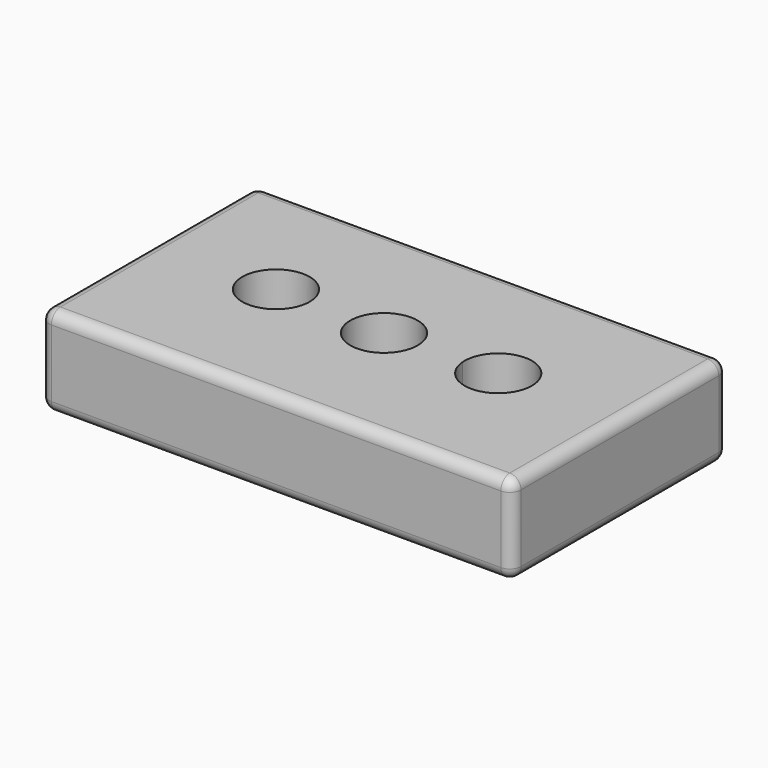
from build123d import *

# Parameters (mm, degrees)
F0_W        = 105
F0_H        = 60
F1_DEPTH    = 20
F2_R        = 2.5
F3_R        = 2.5
F4_R        = 2.5
F5_T1_DEPTH = 23.75
F5_S5_W     = 2.5
F5_S5_H     = 2.5
F5_T6_DEPTH = 2.5
F6_R        = 2.5


# Not quite as in the source:
# - a fillet or chamfer that OpenCascade refuses, or shapes differently, is made with other operations: its cross-section is extruded or revolved along the edge and cut away or added


with BuildPart() as f1:
    # F0 (on Top) → F1 (new body)
    with BuildSketch(Plane.XY):
        Rectangle(F0_W, F0_H)
        with BuildLine():
            ThreePointArc((-17.4192723763, 1.0974504119), (-17.4394815095, 0.547242643), (-17.5, 0))
            ThreePointArc((-17.5, 0), (-32.3990632431, 1.6476581808), (-17.4192723763, 1.0974504119))
        make_face(mode=Mode.SUBTRACT)
        with BuildLine():
            ThreePointArc((-7.5, 0), (0, 7.5), (7.5, 0))
            ThreePointArc((7.5, 0), (0, -7.5), (-7.5, 0))
        make_face(mode=Mode.SUBTRACT)
        with BuildLine():
            ThreePointArc((32.4798090562, 0.5499604379), (25.2549745325, -6.9449901264), (17.5, 0))
            ThreePointArc((17.5, 0), (24.7046435799, 8.0449110021), (32.4798090562, 0.5499604379))
        make_face(mode=Mode.SUBTRACT)
    extrude(amount=F1_DEPTH)

    # F2
    f2_edges = [f1.edges().sort_by_distance(p)[0] for p in [
        (0, -30, 20),
    ]]
    fillet(f2_edges, radius=F2_R)

    # F3
    f3_edges = [f1.edges().sort_by_distance(p)[0] for p in [
        (52.5, 1.25, 20),
        (0, 30, 20),
    ]]
    fillet(f3_edges, radius=F3_R)

    # F4
    f4_edges = [f1.edges().sort_by_distance(p)[0] for p in [
        (-52.5, 0, 20),
    ]]
    fillet(f4_edges, radius=F4_R)

    # F5: fillet of radius 2.5 on 1 edges, made by hand

    # F5_s2 → F5_t1 (cut)
    with BuildSketch(Plane.XY.offset(-6.25)):
        with BuildLine():
            ThreePointArc((50, 30), (51.767766953, 29.267766953), (52.5, 27.5))
            Line((52.5, 27.5), (52.5, 30))
            Line((52.5, 30), (50, 30))
        make_face()
    extrude(amount=F5_T1_DEPTH, mode=Mode.SUBTRACT)


with BuildPart() as f5_tool4:
    # F5_s5 → F5_t6 (new body)
    with BuildSketch(Plane.XZ.offset(-27.5)):
        with Locations((51.25, 18.75)):
            Rectangle(F5_S5_W, F5_S5_H)
    extrude(amount=-F5_T6_DEPTH)

    # F5_s7 → F5_t8 (revolve, cut)
    with BuildSketch(Plane(origin=(50, 27.5, 17.5), x_dir=(-0.7071067812, 0, -0.7071067812), z_dir=(0.7071067812, 0, -0.7071067812))):
        with BuildLine():
            ThreePointArc((0, -2.5), (2.5, 0), (0, 2.5))
            Line((0, 2.5), (0, -2.5))
        make_face()
    revolve(axis=Axis((50, 27.5, 17.5), (0, 1, 0)), mode=Mode.SUBTRACT)


with BuildPart() as f1_1:
    add(f1.part)

    # F5_t3: cut F5_tool4
    add(f5_tool4.part, mode=Mode.SUBTRACT)

    # F6
    f6_edges = [f1_1.edges().sort_by_distance(p)[0] for p in [
        (52.5, 0, 0),
    ]]
    fillet(f6_edges, radius=F6_R)


solid = f1_1.part
